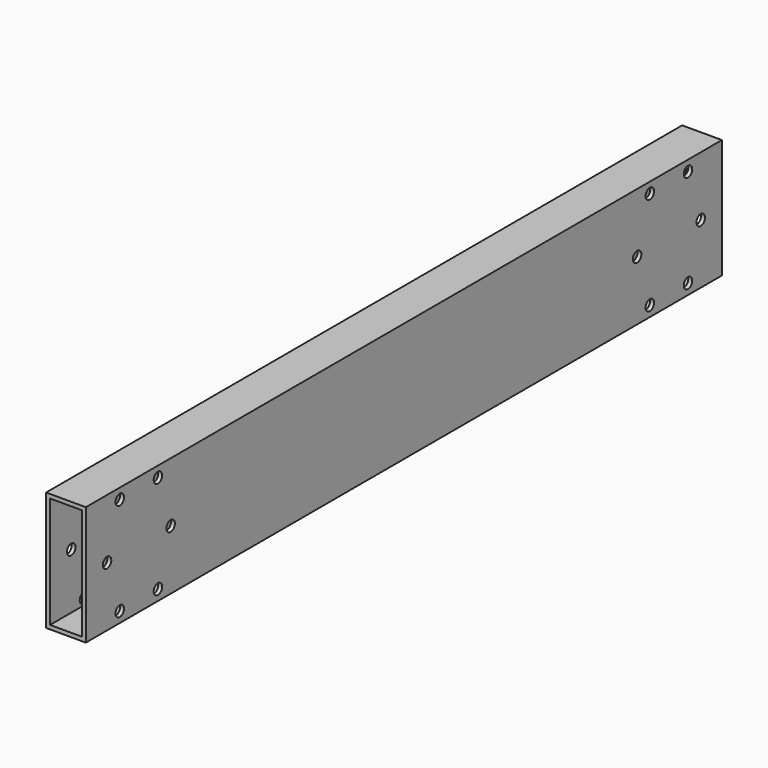
from build123d import *

# Parameters (mm, degrees)
F0_W     = 30
F0_H     = 90
F1_DEPTH = 300
F2_T     = -3
F3_R     = 4
F4_DEPTH = 30.001
F7_R     = 4
F8_DEPTH = 30.001


# Not quite as in the source:
# - a pattern or mirror of a feature is missing from the dataset's text; its kind, count and spacing are read off the source's solid


with BuildPart() as f1:
    # F0 (on Front) → F1 (new body, symmetric)
    with BuildSketch(Plane.XZ):
        Rectangle(F0_W, F0_H)
    extrude(amount=F1_DEPTH, both=True)

    # F2
    f2_openings = [f1.faces().sort_by_distance(p)[0] for p in [
        (0, -300, 0),
        (0, 300, 0),
    ]]
    offset(amount=F2_T, openings=f2_openings)

    # F3 (on face) → F4 (cut, through all)
    with BuildSketch(Plane.YZ.offset(15)):
        with Locations((-268, 37)):
            Circle(F3_R)
        with Locations((-280, 0)):
            Circle(F3_R)
        with Locations((-268, -37)):
            Circle(F3_R)
    f4 = extrude(amount=-F4_DEPTH, mode=Mode.SUBTRACT)

    # F4_copies: F4 across plane
    add(f4.mirror(Plane.ZX.offset(-250)), mode=Mode.SUBTRACT)

    # F7 (on face) → F8 (cut, through all)
    with BuildSketch(Plane.YZ.offset(15)):
        with Locations((268, 37)):
            Circle(F7_R)
        with Locations((280, 0)):
            Circle(F7_R)
        with Locations((268, -37)):
            Circle(F7_R)
    f8 = extrude(amount=-F8_DEPTH, mode=Mode.SUBTRACT)

    # F8_copies: F8 across plane
    add(f8.mirror(Plane(origin=(0, 250, 0), x_dir=(0, 0, -1), z_dir=(0, -1, 0))), mode=Mode.SUBTRACT)


solid = f1.part
